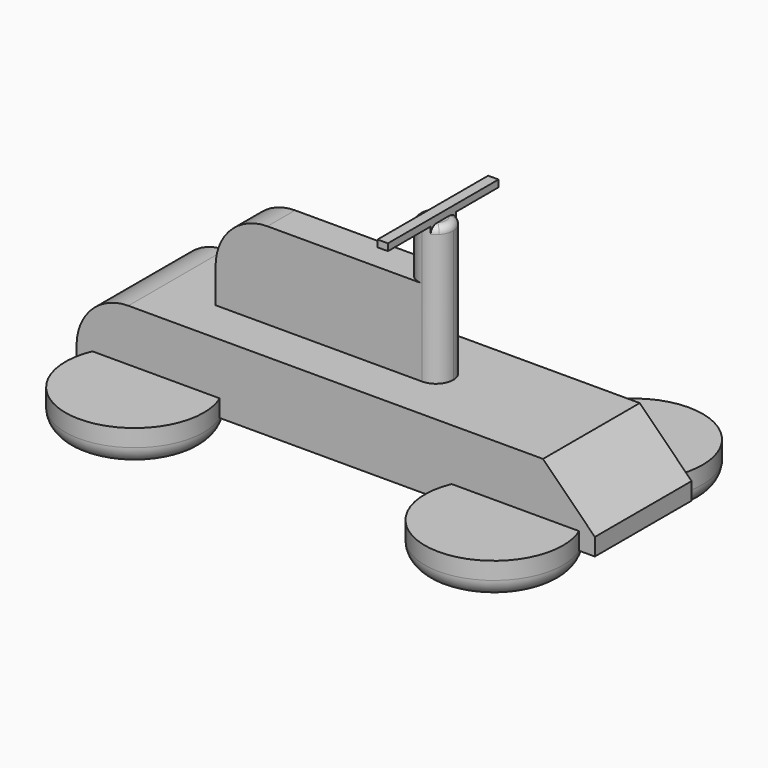
from build123d import *

# Parameters (mm, degrees)
F0_W          = 150
F0_H          = 35
F1_DEPTH      = 10
F3_R          = 20
F4_DEPTH      = 5
F5_R          = 15
F6_SIZE       = 15
F7_R          = 4.99999
F10_DEPTH     = 40
F11_DEPTH     = 25
F12_R         = 15
F14_W         = 3
F14_H         = 40
F15_DEPTH     = 2
F16_T3_ANGLE  = 273.8677552215
F16_T7_ANGLE  = 273.8677552215
F16_T11_ANGLE = 245.1581434466
F16_T15_ANGLE = 245.1581434466


# Not quite as in the source:
# - a fillet or chamfer that OpenCascade refuses, or shapes differently, is made with other operations: its cross-section is extruded or revolved along the edge and cut away or added
# - a fillet or chamfer is up to 0.001 mm smaller than in the source, because OpenCascade refuses the exact size


with BuildPart() as f1:
    # F0 (on Top) → F1 (new body, symmetric)
    with BuildSketch(Plane.XY):
        Rectangle(F0_W, F0_H)
    extrude(amount=F1_DEPTH, both=True)

    # F3 (on offset) → F4 (join, symmetric)
    with BuildSketch(Plane.XY.offset(-10)):
        with Locations((-52, -25.2603590488)):
            Circle(F3_R)
        with Locations((52, -25.2603590488)):
            Circle(F3_R)
        with Locations((52, 25.2603590488)):
            Circle(F3_R)
        with Locations((-52, 25.2603590488)):
            Circle(F3_R)
    extrude(amount=F4_DEPTH, both=True)

    # F5
    f5_edges = [f1.edges().sort_by_distance(p)[0] for p in [
        (-75, 0, 10),
    ]]
    fillet(f5_edges, radius=F5_R)

    # F6
    f6_edges = [f1.edges().sort_by_distance(p)[0] for p in [
        (75, 0, 10),
    ]]
    chamfer(f6_edges, length=F6_SIZE)

    # F7 (radius 5 in the source; OpenCascade refuses exactly that, so slightly less here)
    f7_edges = [f1.edges().sort_by_distance(p)[0] for p in [
        (32, -25.260359, -15),
        (32, 25.260359, -15),
        (-72, -25.260359, -15),
        (-72, 25.260359, -15),
    ]]
    fillet(f7_edges, radius=F7_R)

    # F9 (on offset) → F10 (join)
    with BuildSketch(Plane.XY.offset(10)):
        with BuildLine():
            ThreePointArc((15.0216268376, 5), (10.0216268376, 0), (15.0216268376, -5))
            ThreePointArc((15.0216268376, -5), (18.5571607435, -3.5355339059), (20.0216268376, 0))
            ThreePointArc((20.0216268376, 0), (18.5571607435, 3.5355339059), (15.0216268376, 5))
        make_face()
    extrude(amount=F10_DEPTH)

    # F9 (on offset) → F11 (join)
    with BuildSketch(Plane.XY.offset(10)):
        with BuildLine():
            Line((-44.7599912546, -5), (15.0216268376, -5))
            ThreePointArc((15.0216268376, -5), (10.0216268376, 0), (15.0216268376, 5))
            Line((15.0216268376, 5), (-44.7599912546, 5))
            Line((-44.7599912546, 5), (-44.7599912546, -5))
        make_face()
    extrude(amount=F11_DEPTH)

    # F12
    f12_edges = [f1.edges().sort_by_distance(p)[0] for p in [
        (-44.759991, 0, 35),
    ]]
    fillet(f12_edges, radius=F12_R)

    # F14 (on offset) → F15 (join)
    with BuildSketch(Plane.XY.offset(50)):
        with Locations((15.6161214935, 0)):
            Rectangle(F14_W, F14_H)
    extrude(amount=F15_DEPTH)

    # F16: fillet of radius 2 on 2 edges, made by hand


with BuildPart() as f16_tool1:
    # F16_s2 → F16_t3 (revolve)
    with BuildSketch(Plane(origin=(7.0041804705, 7.4937067775, 0), x_dir=(0, 0, 1), z_dir=(0.6828419269, 0.7305661522, 0))):
        with BuildLine():
            ThreePointArc((48, 15.9742921192), (49.4142135624, 15.3885056815), (50, 13.9742921192))
            Line((50, 13.9742921192), (50, 15.9742921192))
            Line((50, 15.9742921192), (48, 15.9742921192))
        make_face()
    revolve(axis=Axis((15.0216268376, 0, 50), (0, 0, -1)), revolution_arc=F16_T3_ANGLE)

    split(bisect_by=Plane.YZ.offset(17.1161214935), keep=Keep.TOP)


with BuildPart() as f16_tool5:
    # F16_s6 → F16_t7 (revolve)
    with BuildSketch(Plane(origin=(7.0041804705, 7.4937067775, 0), x_dir=(0, 0, 1), z_dir=(0.6828419269, 0.7305661522, 0))):
        with BuildLine():
            ThreePointArc((48, 15.9742921192), (49.4142135624, 15.3885056815), (50, 13.9742921192))
            Line((50, 13.9742921192), (50, 15.9742921192))
            Line((50, 15.9742921192), (48, 15.9742921192))
        make_face()
    revolve(axis=Axis((15.0216268376, 0, 50), (0, 0, -1)), revolution_arc=F16_T7_ANGLE)

    split(bisect_by=Plane.YZ.offset(14.1161214935), keep=Keep.BOTTOM)


with BuildPart() as f16_tool9:
    # F16_s10 → F16_t11 (revolve)
    with BuildSketch(Plane(origin=(10.6662198, 6.8158439522, 0), x_dir=(0, 0, 1), z_dir=(-0.8426491362, -0.5384630287, 0))):
        with BuildLine():
            ThreePointArc((48, -3.0885906834), (49.4142135624, -3.674377121), (50, -5.0885906834))
            Line((50, -5.0885906834), (50, -3.0885906834))
            Line((50, -3.0885906834), (48, -3.0885906834))
        make_face()
    revolve(axis=Axis((15.0216268376, 0, 50), (0, 0, -1)), revolution_arc=F16_T11_ANGLE)

    split(bisect_by=Plane.YZ.offset(14.1161214935), keep=Keep.BOTTOM)


with BuildPart() as f16_tool13:
    # F16_s14 → F16_t15 (revolve)
    with BuildSketch(Plane(origin=(10.6662198, 6.8158439522, 0), x_dir=(0, 0, 1), z_dir=(-0.8426491362, -0.5384630287, 0))):
        with BuildLine():
            ThreePointArc((48, -3.0885906834), (49.4142135624, -3.674377121), (50, -5.0885906834))
            Line((50, -5.0885906834), (50, -3.0885906834))
            Line((50, -3.0885906834), (48, -3.0885906834))
        make_face()
    revolve(axis=Axis((15.0216268376, 0, 50), (0, 0, -1)), revolution_arc=F16_T15_ANGLE)

    split(bisect_by=Plane.YZ.offset(17.1161214935), keep=Keep.TOP)


with BuildPart() as f1_1:
    add(f1.part)

    # F16_t17: cut F16_tool1, F16_tool5, F16_tool9, F16_tool13
    add([f16_tool1.part, f16_tool5.part, f16_tool9.part, f16_tool13.part], mode=Mode.SUBTRACT)


solid = f1_1.part
